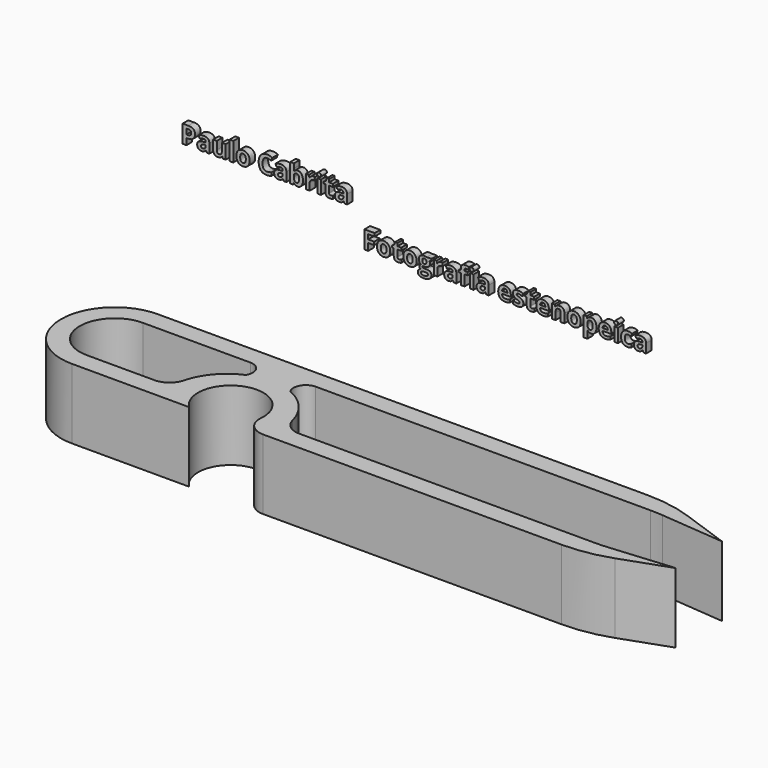
from build123d import *

# Parameters (mm, degrees)
F1_DEPTH     = 7.5
F3_DEPTH     = 7.5
F5_T1_DEPTH  = 15
F5_T3_DEPTH  = 40.7772359705
F6_TEXT_SIZE = 5.3470127743
F7_DEPTH     = 1.5
F8_TEXT_SIZE = 5.3470127743
F9_DEPTH     = 1.5


# Not quite as in the source:
# - a fillet or chamfer that OpenCascade refuses, or shapes differently, is made with other operations: its cross-section is extruded or revolved along the edge and cut away or added
# - a feature names something its author has since deleted; it is built from what else it names
# - Text() gives the source's letters only with a copy of the font that has no kerning and outlines rounded to 1/6400 em; it was checked with that copy


with BuildPart() as f1:
    # F0 (on Top) → F1 (new body, symmetric)
    with BuildSketch(Plane.XY):
        with BuildLine():
            ThreePointArc((-40.9544511501, -7.5), (-48.4544511501, 0), (-40.9544511501, 7.5))
            Line((-40.9544511501, 7.5), (69.0455488499, 7.5))
            Line((69.0455488499, 7.5), (84.0455488499, 6.1876700471))
            Line((84.0455488499, 6.1876700471), (69.0455488499, 11.5))
            Line((69.0455488499, 11.5), (-40.9544511501, 11.5))
            ThreePointArc((-40.9544511501, 11.5), (-52.4544511501, 0), (-40.9544511501, -11.5))
            Line((-40.9544511501, -11.5), (-15.8534306357, -11.5))
            ThreePointArc((-15.8534306357, -11.5), (-13.3697487958, 0.0701093813), (-3.9834367819, -7.1363636364))
            ThreePointArc((-3.9834367819, -7.1363636364), (-2.9541957835, -10.1967994499), (0, -11.5))
            Line((0, -11.5), (69.0455488499, -11.5))
            Line((69.0455488499, -11.5), (84.0455488499, -6.1876700471))
            Line((84.0455488499, -6.1876700471), (69.0455488499, -7.5))
            Line((69.0455488499, -7.5), (4.5374822347, -7.5))
            ThreePointArc((4.5374822347, -7.5), (2.0879924919, -6.6622776602), (0.6644988885, -4.5))
            ThreePointArc((0.6644988885, -4.5), (-10.9544511501, 4.5), (-22.5734011887, -4.5))
            ThreePointArc((-22.5734011887, -4.5), (-23.9968947921, -6.6622776602), (-26.4463845349, -7.5))
            Line((-26.4463845349, -7.5), (-40.9544511501, -7.5))
        make_face()
    extrude(amount=F1_DEPTH, both=True)

    # F2 (on Top) → F3 (join, symmetric)
    with BuildSketch(Plane.XY):
        with BuildLine():
            ThreePointArc((-3.9544511501, 2.2467943448), (-6.5810539777, 4.8733971724), (-3.9544511501, 7.5))
            Line((-3.9544511501, 7.5), (-17.9544511501, 7.5))
            ThreePointArc((-17.9544511501, 7.5), (-15.3278483225, 4.8733971724), (-17.9544511501, 2.2467943448))
            Line((-17.9544511501, 2.2467943448), (-3.9544511501, 2.2467943448))
        make_face()
    extrude(amount=F3_DEPTH, both=True)

    # F5: fillet of radius 30 on 4 edges, made by hand

    # F5_s2 → F5_t1 (join)
    with BuildSketch(Plane.XY.offset(-7.5)):
        with BuildLine():
            ThreePointArc((67.7357205626, -7.5), (69.0443021836, -7.4714466475), (70.3503928451, -7.3858409428))
            Line((70.3503928451, -7.3858409428), (69.0455488499, -7.5))
            Line((69.0455488499, -7.5), (67.7357205626, -7.5))
        make_face()
        with BuildLine():
            ThreePointArc((70.3503928451, 7.3858409428), (69.0443021836, 7.4714466475), (67.7357205626, 7.5))
            Line((67.7357205626, 7.5), (69.0455488499, 7.5))
            Line((69.0455488499, 7.5), (70.3503928451, 7.3858409428))
        make_face()
    extrude(amount=F5_T1_DEPTH)

    # F5_s4 → F5_t3 (cut)
    with BuildSketch(Plane.XY.offset(-20.3886179852)):
        with BuildLine():
            ThreePointArc((63.8901016558, -11.5), (68.9710696165, -11.0665987997), (73.9052310697, -9.7789176388))
            Line((73.9052310697, -9.7789176388), (69.0455488499, -11.5))
            Line((69.0455488499, -11.5), (63.8901016558, -11.5))
        make_face()
        with BuildLine():
            ThreePointArc((73.9052310697, 9.7789176388), (68.9710696165, 11.0665987997), (63.8901016558, 11.5))
            Line((63.8901016558, 11.5), (69.0455488499, 11.5))
            Line((69.0455488499, 11.5), (73.9052310697, 9.7789176388))
        make_face()
    extrude(amount=F5_T3_DEPTH, mode=Mode.SUBTRACT)

    # F6 (on face) → F7 (cut)
    with BuildSketch(Plane(origin=(0, 11.5, 0), x_dir=(-1, 0, 0), z_dir=(0, 1, 0))):
        with Locations((-61.4678252528, 2.5)):
            Text('Paulo Cabrita', F6_TEXT_SIZE, font='Open Sans', font_style=FontStyle.BOLD, text_align=(TextAlign.LEFT, TextAlign.BOTTOM))
        with Locations((-22.5649654365, -4.7719373731)):
            Text('Fotografia estenopeica', F6_TEXT_SIZE, font='Open Sans', font_style=FontStyle.BOLD, text_align=(TextAlign.LEFT, TextAlign.BOTTOM))
    extrude(amount=-F7_DEPTH, mode=Mode.SUBTRACT)


with BuildPart() as f9:
    # F8 (on Front) → F9 (new body)
    with BuildSketch(Plane.XZ):
        with Locations((-25.7044548434, 50)):
            Text('Paulo Cabrita', F8_TEXT_SIZE, font='Open Sans', font_style=FontStyle.BOLD, text_align=(TextAlign.LEFT, TextAlign.BOTTOM))
        with Locations((13.198404973, 42.7280626269)):
            Text('Fotografia estenopeica', F8_TEXT_SIZE, font='Open Sans', font_style=FontStyle.BOLD, text_align=(TextAlign.LEFT, TextAlign.BOTTOM))
    extrude(amount=F9_DEPTH)


solid = Compound([f1.part, f9.part])
